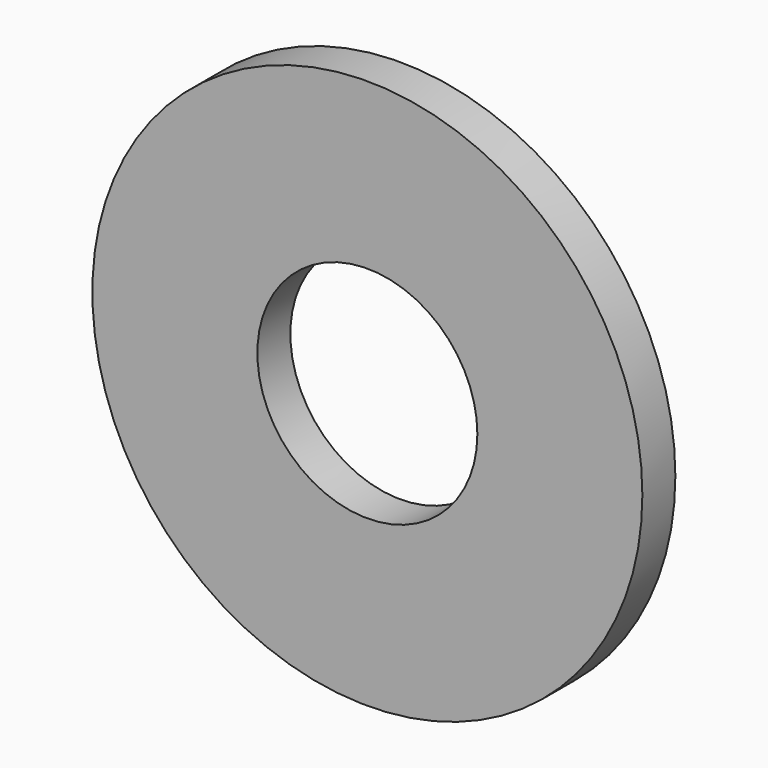
from build123d import *

# Parameters (mm, degrees)
F0_R     = 63.5
F0_R_2   = 25.4
F1_DEPTH = 9.525


# Not quite as in the source:
# - a length typed as a fraction of an inch, garbled in the dataset ("3 / 203.2 mm" for 3/8 in), is restored


with BuildPart() as f1:
    # F0 (on Front) → F1 (new body)
    with BuildSketch(Plane.XZ):
        Circle(F0_R)
        Circle(F0_R_2, mode=Mode.SUBTRACT)
    extrude(amount=F1_DEPTH)


solid = f1.part
